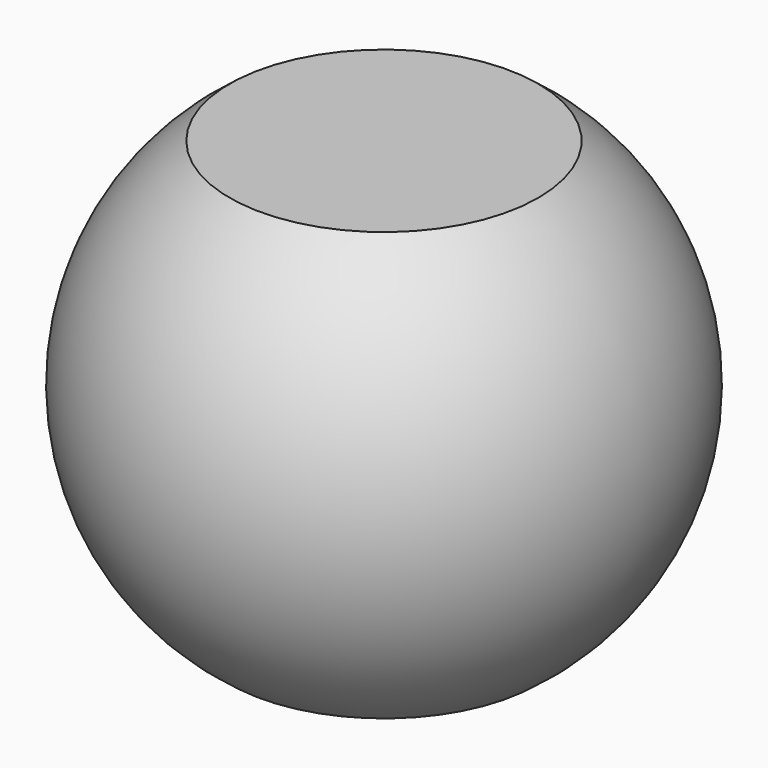
from build123d import *

# Parameters (mm, degrees)
F2_W          = 259.588
F2_H          = 37.084
F3_DEPTH      = 114.301
F3_DEPTH_BACK = 114.301


with BuildPart() as f1:
    # F0 (on Front) → F1 (revolve)
    with BuildSketch(Plane.XZ):
        with BuildLine():
            Line((0, 114.3), (0, -114.3))
            ThreePointArc((0, -114.3), (114.3, 0), (0, 114.3))
        make_face()
    revolve(axis=Axis((0, 0, 0), (0, 0, -1)))

    # F2 (on Front) → F3 (cut, two sides)
    with BuildSketch(Plane.XZ) as f3_sk:
        with Locations((0, 111.252)):
            Rectangle(F2_W, F2_H)
        with Locations((0, -111.252)):
            Rectangle(F2_W, F2_H)
    extrude(amount=-F3_DEPTH, mode=Mode.SUBTRACT)
    extrude(f3_sk.sketch, amount=F3_DEPTH_BACK, mode=Mode.SUBTRACT)


solid = f1.part
